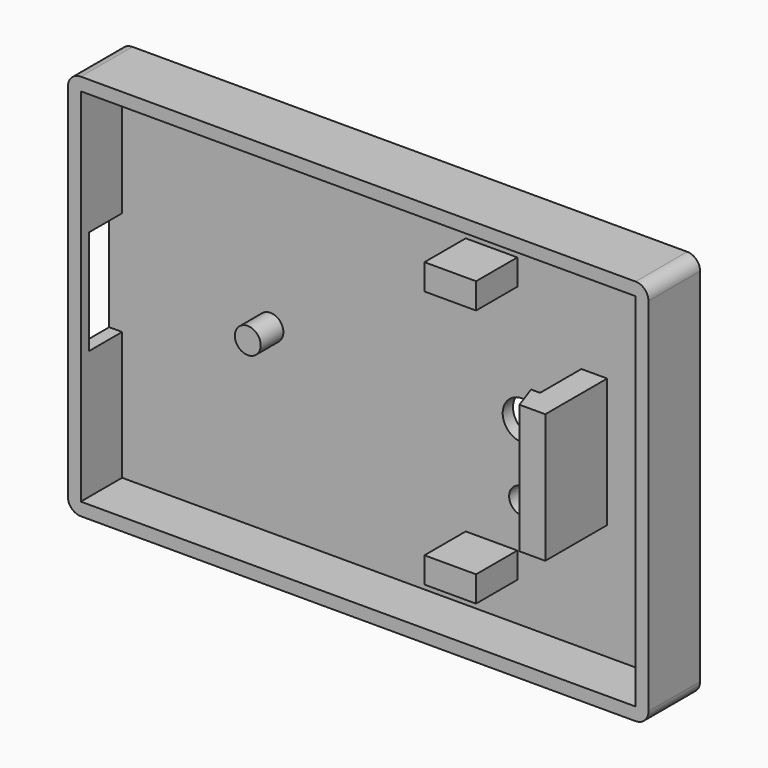
from build123d import *

# Parameters (mm, degrees)
F0_W      = 45
F0_H      = 30
F0_R      = 1
F0_R_2    = 1.5
F1_DEPTH  = 5
F2_R      = 1
F3_T      = 1
F4_W      = 3.2
F4_H      = 8.1
F5_DEPTH  = 25
F6_R      = 1
F7_DEPTH  = 2.2
F10_DEPTH = 5
F11_R     = 0.75
F12_DEPTH = 2.2
F13_W     = 4
F13_H     = 2
F14_DEPTH = 4


# Not quite as in the source:
# - a shell that OpenCascade refuses in one call is made with other operations: the cavity is built on its own and cut out


with BuildPart() as f1:
    # F0 (on Front) → F1 (new body)
    with BuildSketch(Plane.XZ):
        Rectangle(F0_W, F0_H)
        with Locations((9.5, -5.5)):
            Circle(F0_R, mode=Mode.SUBTRACT)
        with Locations((-10, 0)):
            Circle(F0_R, mode=Mode.SUBTRACT)
        with Locations((9.5, 0)):
            Circle(F0_R_2, mode=Mode.SUBTRACT)
        with Locations((-10, 0)):
            Circle(F0_R)
    extrude(amount=F1_DEPTH)

    # F2
    f2_edges = [f1.edges().sort_by_distance(p)[0] for p in [
        (-22.5, -2.5, -15),
        (22.5, -2.5, -15),
        (22.5, -2.5, 15),
        (-22.5, -2.5, 15),
    ]]
    fillet(f2_edges, radius=F2_R)

    # F3: shell of thickness 1, made by hand


with BuildPart() as f3_core1:
    # F3_t2: copy of F1
    add(f1.part)

    # the walls: a layer under each face that stays
    f3_faces = [f3_core1.faces().sort_by_distance(p)[0] for p in [
        (0, -2.5, -15),
        (0, 0, 0),
        (-22.5, -2.5, 0),
        (22.5, -2.5, 0),
        (0, -2.5, 15),
    ]]
    thicken(f3_faces, amount=-F3_T, mode=Mode.SUBTRACT)


with BuildPart() as f1_1:
    add(f1.part)

    # what is left inside the walls is the cavity
    f3_cavity = [f3_core1.part.solids().sort_by_distance(p)[0] for p in [
        (0, -1.01, -4.666667),
    ]]
    add(f3_cavity, mode=Mode.SUBTRACT)

    # F4 (on face) → F5 (cut)
    with BuildSketch(Plane.YZ.offset(-21.5)):
        with Locations((-2.6, 0)):
            Rectangle(F4_W, F4_H)
    extrude(amount=-F5_DEPTH, mode=Mode.SUBTRACT)

    # F6 (on face) → F7 (join)
    with BuildSketch(Plane.XZ.offset(1)):
        with Locations((-10, 0)):
            Circle(F6_R)
    extrude(amount=F7_DEPTH)

    # F9 (on Top) → F10 (join, symmetric)
    with BuildSketch(Plane.XY):
        Polygon((16.1, 0), (14.1, 0), (14.1, -5), (13.4, -5), (14.1, -7), (16.1, -7), align=None)
    extrude(amount=F10_DEPTH, both=True)

    # F11 (on face) → F12 (join, through all)
    with BuildSketch(Plane.XZ.offset(1)):
        with Locations((12.5, 0)):
            Circle(F11_R)
    extrude(amount=F12_DEPTH)

    # F13 (on face) → F14 (join, through all)
    with BuildSketch(Plane.XZ.offset(1)):
        with Locations((7.1361453363, 10)):
            Rectangle(F13_W, F13_H)
        with Locations((7.1361453363, -10)):
            Rectangle(F13_W, F13_H)
    extrude(amount=F14_DEPTH)


solid = f1_1.part
